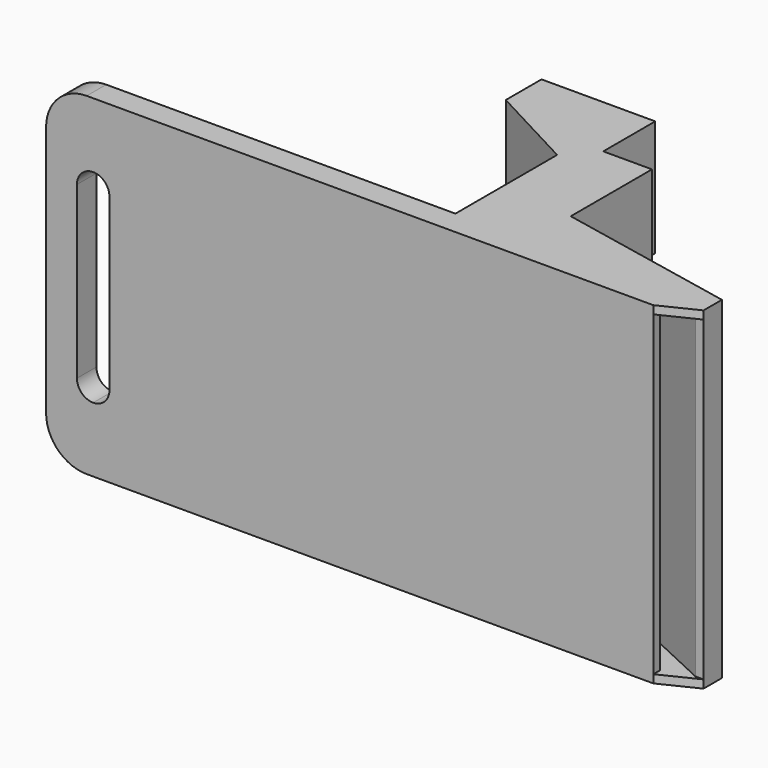
from build123d import *

# Parameters (mm, degrees)
F1_DEPTH  = 39
F3_DEPTH  = 1
F5_DEPTH  = 1
F6_W      = 3
F6_H      = 41
F7_DEPTH  = 48
F8_W      = 4
F8_H      = 25
F9_DEPTH  = 30.001
F10_R     = 1.99999
F11_R     = 5
F12_W     = 15.2
F12_H     = 19.7
F13_DEPTH = 3
F15_DEPTH = 2
F17_DEPTH = 41
F19_DEPTH = 25
F21_DEPTH = 41


# Not quite as in the source:
# - a fillet or chamfer is up to 0.001 mm smaller than in the source, because OpenCascade refuses the exact size
# - ends of sketch curves that miss each other by under 0.0002 mm in the source are joined


with BuildPart() as f1:
    # F0 (on Top) → F1 (new body)
    with BuildSketch(Plane.XY):
        Polygon((0, -8), (0, 0), (-3, 0), (-3, -30), (23.763641715, -30), (23.763641715, -29), (-2, -29), (-2, -9), (0, -9), (4.8176753794, -21.2806219141), (5.7998719041, -21.4797707681), (19.5929166818, -24.2767604715), (27.2138139009, -27.8326366097), (28.2138139009, -27.8326366097), (28.2138139009, -25.9040332723), (28.2138139009, -25.0045752954), (6, -20.5), (6, -8), align=None)
    extrude(amount=F1_DEPTH)

    # F2 (on face) → F3 (join)
    with BuildSketch(Plane.XY.offset(39)):
        Polygon((0, 0), (-3, 0), (-3, -30), (23.763641715, -30), (28.2138139009, -27.8326366097), (28.2138139009, -25.0045752954), (6, -20.5), (6, -8), (0, -8), align=None)
    extrude(amount=F3_DEPTH)

    # F4 (on face) → F5 (join)
    with BuildSketch(Plane(origin=(0, 0, 0), x_dir=(1, 0, 0), z_dir=(0, 0, -1))):
        Polygon((-3, 0), (0, 0), (0, 8), (6, 8), (6, 20.5), (28.2138139009, 25.0045752954), (28.2138139009, 27.8326366097), (23.763641715, 30), (-3, 30), align=None)
    extrude(amount=F5_DEPTH)

    # F6 (on face) → F7 (join)
    with BuildSketch(Plane(origin=(-3, 0, 0), x_dir=(0, -1, 0), z_dir=(-1, 0, 0))):
        with Locations((28.5, 19.5)):
            Rectangle(F6_W, F6_H)
    extrude(amount=F7_DEPTH)

    # F8 (on face) → F9 (cut, through all)
    with BuildSketch(Plane.XZ.offset(30)):
        with Locations((-45.2, 19.5)):
            Rectangle(F8_W, F8_H)
    extrude(amount=-F9_DEPTH, mode=Mode.SUBTRACT)

    # F10 (radius 2 in the source; OpenCascade refuses exactly that, so slightly less here)
    f10_edges = [f1.edges().sort_by_distance(p)[0] for p in [
        (-47.2, -28.5, 32),
        (-43.2, -28.5, 32),
        (-47.2, -28.5, 7),
        (-43.2, -28.5, 7),
    ]]
    fillet(f10_edges, radius=F10_R)

    # F11
    f11_edges = [f1.edges().sort_by_distance(p)[0] for p in [
        (-51, -28.5, 40),
        (-51, -28.5, -1),
    ]]
    fillet(f11_edges, radius=F11_R)

    # F12 (on face) → F13 (cut)
    with BuildSketch(Plane(origin=(-3, 0, 0), x_dir=(0, -1, 0), z_dir=(-1, 0, 0))):
        with Locations((19.4, 19.5)):
            Rectangle(F12_W, F12_H)
    extrude(amount=-F13_DEPTH, mode=Mode.SUBTRACT)

    # F14 (on face) → F15 (join)
    with BuildSketch(Plane(origin=(-3, 0, 0), x_dir=(0, -1, 0), z_dir=(-1, 0, 0))):
        Polygon((10.8, 30.35), (10.8, 8.65), (27, 8.65), (27, 9.65), (11.8, 9.65), (11.8, 29.35), (27, 29.35), (27, 30.35), align=None)
    extrude(amount=-F15_DEPTH)

    # F16 (on face) → F17 (join, through all)
    with BuildSketch(Plane(origin=(0, 0, -1), x_dir=(1, 0, 0), z_dir=(0, 0, -1))):
        Polygon((-14, 0), (-3, 0), (-3, 8), (-14, 5.5), align=None)
    extrude(amount=-F17_DEPTH)

    # F18 (on face) → F19 (cut)
    with BuildSketch(Plane(origin=(-14, 0, 0), x_dir=(0, -1, 0), z_dir=(-1, 0, 0))):
        with BuildLine():
            Line((-0.9789119939, 3.5), (2.125, 3.5))
            ThreePointArc((2.125, 3.5), (4.25, 5.625), (2.125, 7.75))
            Line((2.125, 7.75), (-0.9789119939, 7.75))
            Line((-0.9789119939, 7.75), (-0.9789119939, 3.5))
        make_face()
        with BuildLine():
            Line((-0.98, 21.45), (2.125, 21.45))
            ThreePointArc((2.125, 21.45), (4.25, 23.575), (2.125, 25.7))
            Line((2.125, 25.7), (-0.98, 25.7))
            Line((-0.98, 25.7), (-0.98, 21.45))
        make_face()
    extrude(amount=-F19_DEPTH, mode=Mode.SUBTRACT)

    # F20 (on face) → F21 (join, through all)
    with BuildSketch(Plane.XY.offset(40)):
        Polygon((-3, -8), (-14, -5.5), (-3, -11.3482829183), align=None)
    extrude(amount=-F21_DEPTH)


solid = f1.part
